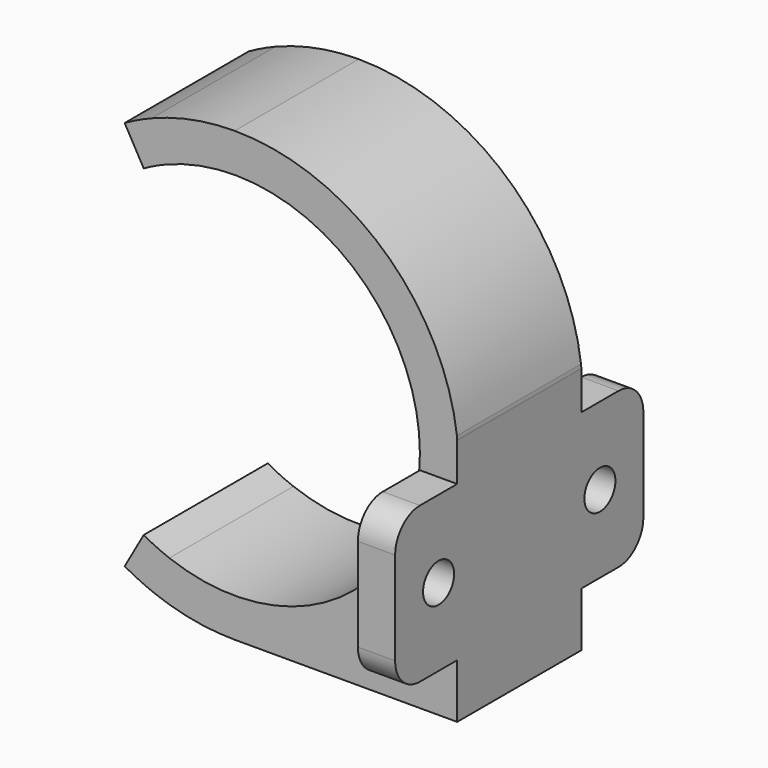
from build123d import *

# Parameters (mm, degrees)
F2_DEPTH = 25.4
F3_W     = 6.096
F3_H     = 50.8
F4_DEPTH = 25.4
F5_R     = 5.08
F6_R     = 3.175
F7_DEPTH = 6.097
F8_R     = 3.175
F9_DEPTH = 6.097


# Not quite as in the source:
# - a feature names something its author has since deleted; it is built from what else it names


with BuildPart() as f2:
    # F1 (on Front) → F2 (new body)
    with BuildSketch(Plane.XZ):
        with BuildLine():
            ThreePointArc((-4.1881381368, 58.1348573723), (-17.2625408115, 33.1930369346), (-45.2129217657, 29.7563791738))
            ThreePointArc((-45.2129217657, 29.7563791738), (-47.3496102258, 30.6565141034), (-49.4112893939, 31.7172494495))
            Line((-49.4112893939, 31.7172494495), (-52.5301234092, 26.1859408896))
            ThreePointArc((-52.5301234092, 26.1859408896), (-50.0367693734, 24.903108528), (-47.4527005825, 23.8145031357))
            ThreePointArc((-47.4527005825, 23.8145031357), (-41.0907281326, 22.0513224192), (-34.5157381367, 21.4571791316))
            Line((-34.5157381367, 21.4571791316), (1.9167693099, 21.4571791316))
            Line((1.9167693099, 21.4571791316), (1.9167693099, 62.3678327477))
            ThreePointArc((1.9167693099, 62.3678327477), (-10.1232383217, 85.5255128665), (-34.5157381367, 94.8123791316))
            ThreePointArc((-34.5157381367, 94.8123791316), (-41.4558425944, 94.1497939431), (-48.145199434, 92.1859777376))
            ThreePointArc((-48.145199434, 92.1859777376), (-50.3725422349, 91.2075489816), (-52.5301234092, 90.0836173735))
            Line((-52.5301234092, 90.0836173735), (-49.4112893939, 84.5523088136))
            ThreePointArc((-49.4112893939, 84.5523088136), (-47.6272506666, 85.4816539244), (-45.7855281567, 86.2906871202))
            ThreePointArc((-45.7855281567, 86.2906871202), (-17.5160993904, 83.2500255818), (-4.1881381368, 58.1348573723))
        make_face()
    extrude(amount=F2_DEPTH)

    # F3 (on offset) → F4 (join)
    with BuildSketch(Plane.XY.offset(30.353)):
        with Locations((-1.1312306901, -12.7)):
            Rectangle(F3_W, F3_H)
    extrude(amount=F4_DEPTH)

    # F5
    f5_edges = [f2.edges().sort_by_distance(p)[0] for p in [
        (1.916769, -12.7, 62.367833),
        (-1.131231, -38.1, 55.753),
        (-1.131231, -38.1, 30.353),
        (-1.131231, 12.7, 30.353),
        (-1.131231, 12.7, 55.753),
    ]]
    fillet(f5_edges, radius=F5_R)

    # F6 (on face) → F7 (cut, through all)
    with BuildSketch(Plane(origin=(-4.1792306901, 0, 0), x_dir=(0, -1, 0), z_dir=(-1, 0, 0))):
        with Locations((-3.81, 43.053)):
            Circle(F6_R)
    extrude(amount=-F7_DEPTH, mode=Mode.SUBTRACT)

    # F8 (on face) → F9 (cut, through all)
    with BuildSketch(Plane(origin=(-4.1792306901, 0, 0), x_dir=(0, -1, 0), z_dir=(-1, 0, 0))):
        with Locations((29.21, 43.053)):
            Circle(F8_R)
    extrude(amount=-F9_DEPTH, mode=Mode.SUBTRACT)


solid = f2.part
